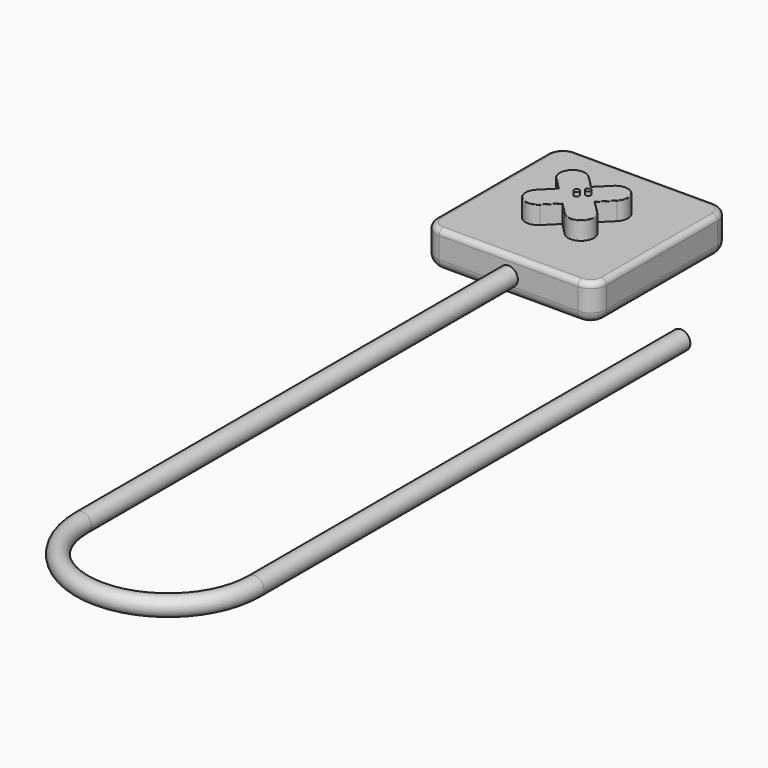
from build123d import *

# Parameters (mm, degrees)
F1_DEPTH     = 7
F3_DEPTH     = 3.4
F5_DEPTH     = 0.74
F6_R         = 1.75
F7_DEPTH     = 3
F8_T1_DEPTH  = 26
F8_T3_DEPTH  = 26
F8_T6_ANGLE  = 90
F8_T8_ANGLE  = 90
F8_T10_ANGLE = 90
F8_T12_ANGLE = 90
F9_R         = 1
F10_R        = 0.1


# Not quite as in the source:
# - a fillet or chamfer that OpenCascade refuses, or shapes differently, is made with other operations: its cross-section is extruded or revolved along the edge and cut away or added


with BuildPart() as f1:
    # F0 (on Top) → F1 (new body)
    with BuildSketch(Plane.XY):
        with BuildLine():
            Line((13, 16), (-13, 16))
            ThreePointArc((-13, 16), (-15.1213203436, 15.1213203436), (-16, 13))
            Line((-16, 13), (-16, -13))
            ThreePointArc((-16, -13), (-15.1213203436, -15.1213203436), (-13, -16))
            Line((-13, -16), (13, -16))
            ThreePointArc((13, -16), (15.1213203436, -15.1213203436), (16, -13))
            Line((16, -13), (16, 13))
            ThreePointArc((16, 13), (15.1213203436, 15.1213203436), (13, 16))
        make_face()
    extrude(amount=F1_DEPTH)

    # F2 (on face) → F3 (join)
    with BuildSketch(Plane.XY.offset(7)):
        with BuildLine():
            Line((0, 3.3941125497), (-2.3029437252, 5.6970562748))
            ThreePointArc((-2.3029437252, 5.6970562748), (-5.6970562748, 5.6970562748), (-5.6970562748, 2.3029437252))
            Line((-5.6970562748, 2.3029437252), (-3.3941125497, 0))
            Line((-3.3941125497, 0), (-5.6970562748, -2.3029437252))
            ThreePointArc((-5.6970562748, -2.3029437252), (-5.6970562748, -5.6970562748), (-2.3029437252, -5.6970562748))
            Line((-2.3029437252, -5.6970562748), (0, -3.3941125497))
            Line((0, -3.3941125497), (2.3029437252, -5.6970562748))
            ThreePointArc((2.3029437252, -5.6970562748), (5.6970562748, -5.6970562748), (5.6970562748, -2.3029437252))
            Line((5.6970562748, -2.3029437252), (3.3941125497, 0))
            Line((3.3941125497, 0), (5.6970562748, 2.3029437252))
            ThreePointArc((5.6970562748, 2.3029437252), (5.6970562748, 5.6970562748), (2.3029437252, 5.6970562748))
            Line((2.3029437252, 5.6970562748), (0, 3.3941125497))
        make_face()
    extrude(amount=F3_DEPTH)

    # F4 (on face) → F5 (join)
    with BuildSketch(Plane.XY.offset(10.4)):
        with BuildLine():
            ThreePointArc((0.3535533906, 0.3535533906), (-0.4619397663, -0.1913417162), (0.5, 0))
            ThreePointArc((0.5, 0), (0.4619397663, 0.1913417162), (0.3535533906, 0.3535533906))
        make_face()
        with BuildLine():
            ThreePointArc((1.5591911551, 1.5591911551), (0.8520843739, 1.5591911551), (0.8520843739, 0.8520843739))
            Line((0.8520843739, 0.8520843739), (1.5591911551, 1.5591911551))
        make_face()
        with BuildLine():
            Line((1.5591911551, 1.5591911551), (0.8520843739, 0.8520843739))
            ThreePointArc((0.8520843739, 0.8520843739), (1.3969794806, 0.7436979982), (1.7056377645, 1.2056377645))
            ThreePointArc((1.7056377645, 1.2056377645), (1.6675775307, 1.3969794806), (1.5591911551, 1.5591911551))
        make_face()
    extrude(amount=F5_DEPTH)

    # F6 (on face) → F7 (cut)
    with BuildSketch(Plane.XZ.offset(16)):
        with Locations((0, 3.5)):
            Circle(F6_R)
    extrude(amount=-F7_DEPTH, mode=Mode.SUBTRACT)

    # F8: fillet of radius 2 on 8 edges, made by hand

    # F8_s2 → F8_t1 (cut)
    with BuildSketch(Plane.YZ.offset(-13)):
        with BuildLine():
            ThreePointArc((-14, 0), (-15.4142135624, 0.5857864376), (-16, 2))
            Line((-16, 2), (-16, 0))
            Line((-16, 0), (-14, 0))
        make_face()
        with BuildLine():
            ThreePointArc((16, 2), (15.4142135624, 0.5857864376), (14, 0))
            Line((14, 0), (16, 0))
            Line((16, 0), (16, 2))
        make_face()
    extrude(amount=F8_T1_DEPTH, mode=Mode.SUBTRACT)

    # F8_s4 → F8_t3 (cut)
    with BuildSketch(Plane.XZ.offset(-13)):
        with BuildLine():
            ThreePointArc((-14, 0), (-15.4142135624, 0.5857864376), (-16, 2))
            Line((-16, 2), (-16, 0))
            Line((-16, 0), (-14, 0))
        make_face()
        with BuildLine():
            ThreePointArc((14, 0), (15.4142135624, 0.5857864376), (16, 2))
            Line((16, 2), (16, 0))
            Line((16, 0), (14, 0))
        make_face()
    extrude(amount=F8_T3_DEPTH, mode=Mode.SUBTRACT)

    # F8_s5 → F8_t6 (revolve, cut)
    with BuildSketch(Plane.XZ.offset(-13)):
        with BuildLine():
            ThreePointArc((16, 2), (15.4142135624, 0.5857864376), (14, 0))
            Line((14, 0), (16, 0))
            Line((16, 0), (16, 2))
        make_face()
    revolve(axis=Axis((13, 13, 0), (0, 0, 1)), revolution_arc=F8_T6_ANGLE, mode=Mode.SUBTRACT)

    # F8_s7 → F8_t8 (revolve, cut)
    with BuildSketch(Plane.YZ.offset(-13)):
        with BuildLine():
            ThreePointArc((16, 2), (15.4142135624, 0.5857864376), (14, 0))
            Line((14, 0), (16, 0))
            Line((16, 0), (16, 2))
        make_face()
    revolve(axis=Axis((-13, 13, 0), (0, 0, 1)), revolution_arc=F8_T8_ANGLE, mode=Mode.SUBTRACT)

    # F8_s9 → F8_t10 (revolve, cut)
    with BuildSketch(Plane.XZ.offset(13)):
        with BuildLine():
            ThreePointArc((-14, 0), (-15.4142135624, 0.5857864376), (-16, 2))
            Line((-16, 2), (-16, 0))
            Line((-16, 0), (-14, 0))
        make_face()
    revolve(axis=Axis((-13, -13, 0), (0, 0, 1)), revolution_arc=F8_T10_ANGLE, mode=Mode.SUBTRACT)

    # F8_s11 → F8_t12 (revolve, cut)
    with BuildSketch(Plane.YZ.offset(13)):
        with BuildLine():
            ThreePointArc((-14, 0), (-15.4142135624, 0.5857864376), (-16, 2))
            Line((-16, 2), (-16, 0))
            Line((-16, 0), (-14, 0))
        make_face()
    revolve(axis=Axis((13, -13, 0), (0, 0, 1)), revolution_arc=F8_T12_ANGLE, mode=Mode.SUBTRACT)

    # F9
    f9_edges = [f1.edges().sort_by_distance(p)[0] for p in [
        (0, -16, 7),
        (-15.12132, 15.12132, 7),
        (-16, 0, 7),
        (0, 16, 7),
        (15.12132, 15.12132, 7),
        (16, 0, 7),
        (15.12132, -15.12132, 7),
        (-15.12132, -15.12132, 7),
    ]]
    fillet(f9_edges, radius=F9_R)

    # F10
    f10_edges = [f1.edges().sort_by_distance(p)[0] for p in [
        (-1.151472, -4.545584, 10.4),
        (1.151472, -4.545584, 10.4),
        (4.545584, 1.151472, 10.4),
        (-1.151472, 4.545584, 10.4),
        (5.697056, 5.697056, 10.4),
        (1.151472, 4.545584, 10.4),
        (-5.697056, 5.697056, 10.4),
        (-4.545584, 1.151472, 10.4),
        (-4.545584, -1.151472, 10.4),
        (-5.697056, -5.697056, 10.4),
        (5.697056, -5.697056, 10.4),
        (4.545584, -1.151472, 10.4),
    ]]
    fillet(f10_edges, radius=F10_R)


with BuildPart() as f12:
    # F12: sweep along a path in F11
    with BuildLine(Plane.XY) as f12_path:
        Line((-1.316445414, -16), (-1.316445414, -116))
        ThreePointArc((-1.316445414, -116), (16.183554586, -133.5), (33.683554586, -116))
        Line((33.683554586, -116), (33.683554586, -16))
    # F6 (on face) → F12 (sweep)
    with BuildSketch(Plane.XZ.offset(16)):
        with Locations((0, 3.5)):
            Circle(F6_R)
    sweep(path=f12_path.line)


solid = Compound([f1.part, f12.part])
